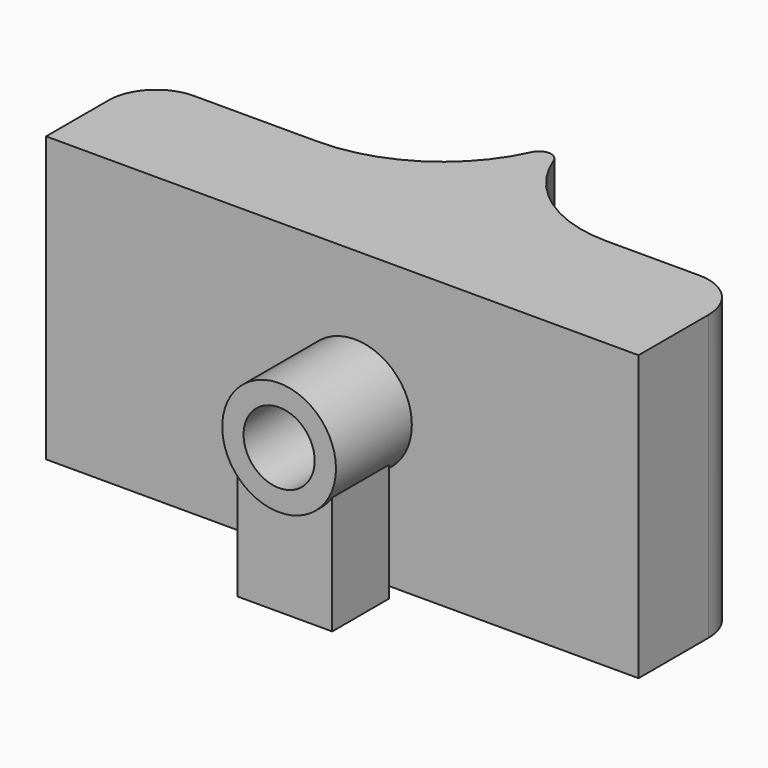
from build123d import *

# Parameters (mm, degrees)
F1_DEPTH = 12
F2_R     = 1.5
F3_DEPTH = 25
F4_R     = 0.5
F5_R     = 2
F2_R_2   = 2.4
F6_DEPTH = 4


# Not quite as in the source:
# - a feature names something its author has since deleted; it is built from what else it names


with BuildPart() as f1:
    # F0 (on Top) → F1 (new body)
    with BuildSketch(Plane.XY):
        with BuildLine():
            Line((12.5, 6.4), (6.5829587897, 6.4))
            ThreePointArc((6.5829587897, 6.4), (2.6961571623, 8.0968384564), (1.2981383552, 12.100840336))
            ThreePointArc((1.2981383552, 12.100840336), (-0.7960029052, 7.7598319357), (-5.2829587897, 6))
            Line((-5.2829587897, 6), (-12.5, 6))
            Line((-12.5, 6), (-12.5, 0.7))
            Line((-12.5, 0.7), (12.5, 0.7))
            Line((12.5, 0.7), (12.5, 6.4))
        make_face()
    extrude(amount=F1_DEPTH)

    # F2 (on face) → F3 (cut)
    with BuildSketch(Plane.XZ.offset(-0.7)):
        with Locations((0.5329587897, 6.3)):
            Circle(F2_R)
    extrude(amount=-F3_DEPTH, mode=Mode.SUBTRACT)

    # F4
    f4_edges = [f1.edges().sort_by_distance(p)[0] for p in [
        (1.298138, 12.10084, 9.795078),
        (1.298138, 12.10084, 2.504922),
    ]]
    fillet(f4_edges, radius=F4_R)

    # F5
    f5_edges = [f1.edges().sort_by_distance(p)[0] for p in [
        (-12.5, 6, 6),
        (12.5, 6.4, 6),
    ]]
    fillet(f5_edges, radius=F5_R)

    # F2 (on face) → F6 (join)
    with BuildSketch(Plane.XZ.offset(-0.7)):
        with Locations((0.5329587897, 6.3)):
            Circle(F2_R_2)
        with Locations((0.5329587897, 6.3)):
            Circle(F2_R, mode=Mode.SUBTRACT)
    extrude(amount=F6_DEPTH)

    # F0 (on Top) → F7 (join, up to the next surface of F1)
    with BuildSketch(Plane.XY):
        Polygon((-0.4670412103, 0), (-1.4670412103, 0), (-1.4670412103, -2), (-1.4670412103, -3), (2.5329587897, -3), (2.5329587897, -2), (2.5329587897, 0), (1.5329587897, 0), (1.5329587897, -2), (-0.4670412103, -2), align=None)
    extrude(until=Until.NEXT)


solid = f1.part
